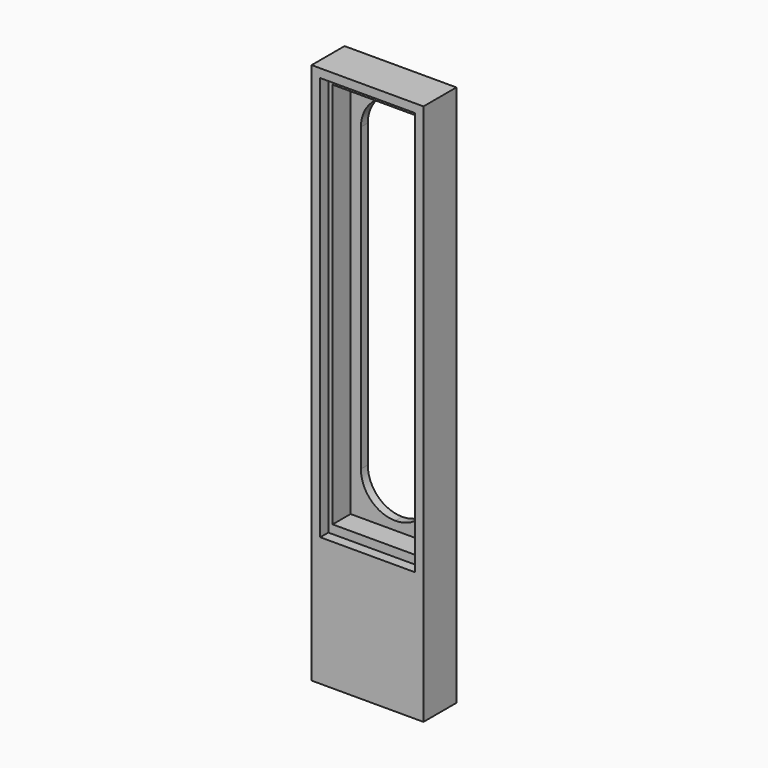
from build123d import *

# Parameters (mm, degrees)
F0_W        = 165.1
F0_H        = 800.1
F0_W_2      = 139.7
F0_H_2      = 596.9
F0_W_3      = 127
F0_H_3      = 571.5
F0_W_4      = 101.6
F0_H_4      = 546.1
F1_DEPTH    = 50.8
F2_DEPTH    = 5
F3_DEPTH    = 38.1
F4_R        = 50.79999
F2_FACE_W   = 165.1
F2_FACE_H   = 800.1
F2_FACE_W_2 = 139.7
F2_FACE_H_2 = 596.9
F5_DEPTH    = 10


# Not quite as in the source:
# - a fillet or chamfer is up to 0.001 mm smaller than in the source, because OpenCascade refuses the exact size
# - a feature names something its author has since deleted; it is built from what else it names


with BuildPart() as f1:
    # F0 (on Front) → F1 (new body)
    with BuildSketch(Plane.XZ):
        with Locations((0, 209.55)):
            Rectangle(F0_W, F0_H)
        with Locations((0, 298.45)):
            Rectangle(F0_W_2, F0_H_2, mode=Mode.SUBTRACT)
        with Locations((0, 298.45)):
            Rectangle(F0_W_2, F0_H_2)
        with Locations((0, 298.45)):
            Rectangle(F0_W_3, F0_H_3, mode=Mode.SUBTRACT)
        with Locations((0, 298.45)):
            Rectangle(F0_W_3, F0_H_3)
        with Locations((2.54, 298.45)):
            Rectangle(F0_W_4, F0_H_4, mode=Mode.SUBTRACT)
    extrude(amount=-F1_DEPTH)

    # F0 (on Front) → F2 (cut)
    with BuildSketch(Plane.XZ):
        with Locations((0, 298.45)):
            Rectangle(F0_W_2, F0_H_2)
        with Locations((0, 298.45)):
            Rectangle(F0_W_3, F0_H_3, mode=Mode.SUBTRACT)
    extrude(amount=-F2_DEPTH, mode=Mode.SUBTRACT)

    # F0 (on Front) → F3 (cut)
    with BuildSketch(Plane.XZ):
        with Locations((0, 298.45)):
            Rectangle(F0_W_3, F0_H_3)
        with Locations((2.54, 298.45)):
            Rectangle(F0_W_4, F0_H_4, mode=Mode.SUBTRACT)
    extrude(amount=-F3_DEPTH, mode=Mode.SUBTRACT)

    # F4 (radius 50.8 in the source; OpenCascade refuses exactly that, so slightly less here)
    f4_edges = [f1.edges().sort_by_distance(p)[0] for p in [
        (53.34, 44.45, 571.5),
        (-48.26, 44.45, 571.5),
        (-48.26, 44.45, 25.4),
        (53.34, 44.45, 25.4),
    ]]
    fillet(f4_edges, radius=F4_R)

    # F0 (on Front) + F2_face (on face) → F5 (join)
    with BuildSketch(Plane.XZ):
        with Locations((0, 209.55)):
            Rectangle(F0_W, F0_H)
        with Locations((0, 298.45)):
            Rectangle(F0_W_2, F0_H_2, mode=Mode.SUBTRACT)
    with BuildSketch(Plane(origin=(0, 0, 57.3602649007), x_dir=(1, 0, 0), z_dir=(0, -1, 0))):
        with Locations((0, 152.1897350993)):
            Rectangle(F2_FACE_W, F2_FACE_H)
        with Locations((0, 241.0897350993)):
            Rectangle(F2_FACE_W_2, F2_FACE_H_2, mode=Mode.SUBTRACT)
    extrude(amount=F5_DEPTH)


solid = f1.part
